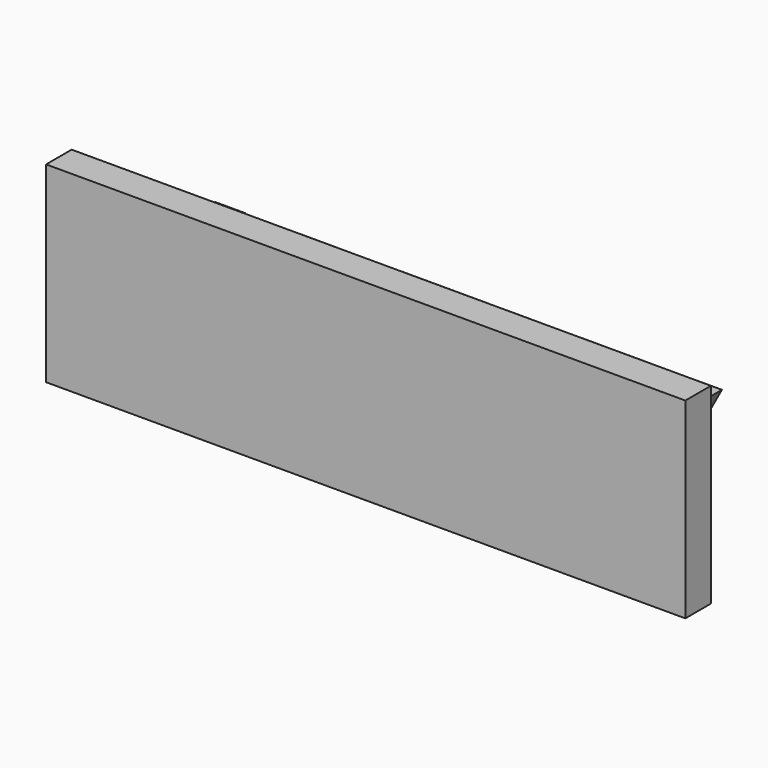
from build123d import *

# Parameters (mm, degrees)
F0_TEXT_SIZE = 10.3449868379
F1_DEPTH     = 3
F2_W         = 40
F2_H         = 12
F3_DEPTH     = 2


# Not quite as in the source:
# - Text() gives the source's letters only with a copy of the font that has no kerning and outlines rounded to 1/6400 em; it was checked with that copy


with BuildPart() as f1:
    # F0 (on Front) → F1 (new body)
    with BuildSketch(Plane.XZ):
        with Locations((-18.000276852, -3.918163948)):
            Text('ARTHY', F0_TEXT_SIZE, font='Open Sans', font_style=FontStyle.BOLD, text_align=(TextAlign.LEFT, TextAlign.BOTTOM))
    extrude(amount=-F1_DEPTH)


with BuildPart() as f3:
    # F2 (on Front) → F3 (new body)
    with BuildSketch(Plane.XZ):
        with Locations((-1.958956942, -0.5358985201)):
            Rectangle(F2_W, F2_H)
    extrude(amount=F3_DEPTH)


solid = Compound([f1.part, f3.part])
